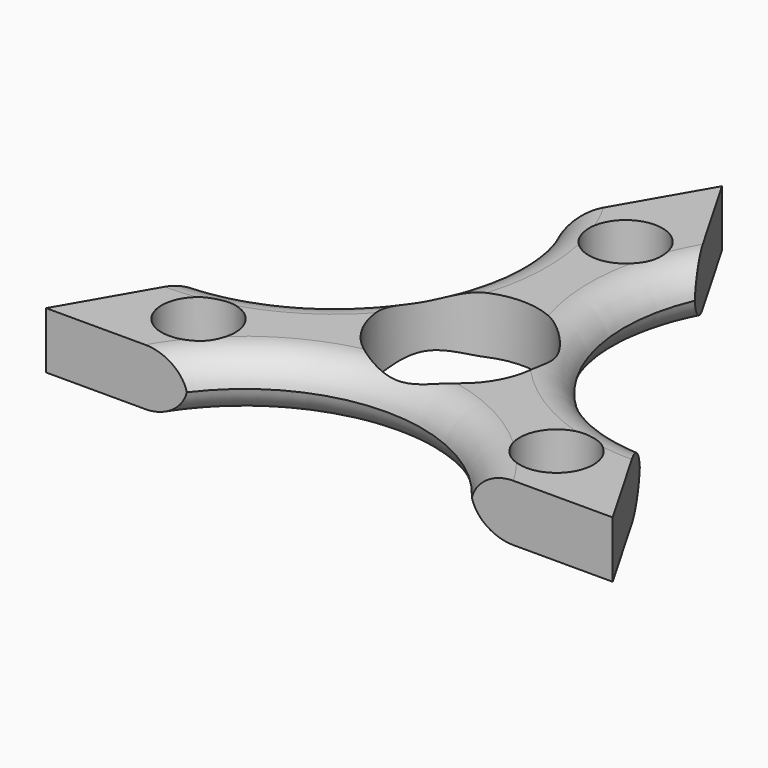
from build123d import *

# Parameters (mm, degrees)
F0_R         = 5.2
F0_R_2       = 11
F1_DEPTH     = 8
F2_T2_ANGLE  = 163.5880718536
F2_T4_ANGLE  = 163.5880718536
F2_T6_ANGLE  = 163.5880718536
F2_T8_ANGLE  = 163.5880718536
F2_T10_ANGLE = 163.5880718536
F2_T12_ANGLE = 163.5880718536


# Not quite as in the source:
# - a fillet or chamfer that OpenCascade refuses, or shapes differently, is made with other operations: its cross-section is extruded or revolved along the edge and cut away or added


with BuildPart() as f1:
    # F0 (on Top) → F1 (new body)
    with BuildSketch(Plane.XY):
        with BuildLine():
            Line((10, 28.4363744997), (0, 45.7568825754))
            Line((0, 45.7568825754), (-10, 28.4363744997))
            ThreePointArc((-10, 28.4363744997), (-11.3397459622, 6.115866424), (-30, -6.2046416517))
            Line((-30, -6.2046416517), (-40, -23.5251497274))
            Line((-40, -23.5251497274), (-20, -23.5251497274))
            ThreePointArc((-20, -23.5251497274), (0, -13.5251497274), (20, -23.5251497274))
            Line((20, -23.5251497274), (40, -23.5251497274))
            Line((40, -23.5251497274), (30, -6.2046416517))
            ThreePointArc((30, -6.2046416517), (11.3397459622, 6.115866424), (10, 28.4363744997))
        make_face()
        with Locations((-25.2775681357, -15.0251497274)):
            Circle(F0_R, mode=Mode.SUBTRACT)
        with Locations((25.2775681357, -15.0251497274)):
            Circle(F0_R, mode=Mode.SUBTRACT)
        with Locations((0, -0.4311389598)):
            Circle(F0_R_2, mode=Mode.SUBTRACT)
        with Locations((0, 28.7568825754)):
            Circle(F0_R, mode=Mode.SUBTRACT)
    extrude(amount=F1_DEPTH)

    # F2: fillet of radius 5 on 6 edges, made by hand

    # F2_s1 → F2_t2 (revolve, cut)
    with BuildSketch(Plane(origin=(-29.4179701652, 23.1546186531, 0), x_dir=(0, 0, 1), z_dir=(-0.7857925171, 0.618490194, 0))):
        with BuildLine():
            ThreePointArc((3, 19.2239813561), (6.5355339059, 20.6884474501), (8, 24.2239813561))
            Line((8, 24.2239813561), (8, 19.2239813561))
            Line((8, 19.2239813561), (3, 19.2239813561))
        make_face()
    revolve(axis=Axis((-32.9903810568, 18.615866424, 8), (0, 0, -1)), revolution_arc=F2_T2_ANGLE, mode=Mode.SUBTRACT)

    # F2_s3 → F2_t4 (revolve, cut)
    with BuildSketch(Plane(origin=(34.8604405257, 13.9389723807, 0), x_dir=(0, 0, 1), z_dir=(0.9285244785, 0.3712711849, 0))):
        with BuildLine():
            ThreePointArc((3, 19.9630902024), (6.5355339059, 21.4275562964), (8, 24.9630902024))
            Line((8, 24.9630902024), (8, 19.9630902024))
            Line((8, 19.9630902024), (3, 19.9630902024))
        make_face()
    revolve(axis=Axis((32.9903810568, 18.615866424, 8), (0, 0, -1)), revolution_arc=F2_T4_ANGLE, mode=Mode.SUBTRACT)

    # F2_s5 → F2_t6 (revolve, cut)
    with BuildSketch(Plane(origin=(-5.4424703605, -37.7402994735, 0), x_dir=(0, 0, 1), z_dir=(-0.1427319614, -0.9897613789, 0))):
        with BuildLine():
            ThreePointArc((3, 19.5012298151), (6.5355339059, 20.9656959092), (8, 24.5012298151))
            Line((8, 24.5012298151), (8, 19.5012298151))
            Line((8, 19.5012298151), (3, 19.5012298151))
        make_face()
    revolve(axis=Axis((0, -38.5251497274, 8), (0, 0, -1)), revolution_arc=F2_T6_ANGLE, mode=Mode.SUBTRACT)

    # F2_s7 → F2_t8 (revolve, cut)
    with BuildSketch(Plane(origin=(-29.4179701652, 23.1546186531, 0), x_dir=(0, 0, 1), z_dir=(-0.7857925171, 0.618490194, 0))):
        with BuildLine():
            ThreePointArc((5, 19.2239813561), (1.4644660941, 20.6884474501), (0, 24.2239813561))
            Line((0, 24.2239813561), (0, 19.2239813561))
            Line((0, 19.2239813561), (5, 19.2239813561))
        make_face()
    revolve(axis=Axis((-32.9903810568, 18.615866424, 0), (0, 0, -1)), revolution_arc=F2_T8_ANGLE, mode=Mode.SUBTRACT)

    # F2_s9 → F2_t10 (revolve, cut)
    with BuildSketch(Plane(origin=(34.8604405257, 13.9389723807, 0), x_dir=(0, 0, 1), z_dir=(0.9285244785, 0.3712711849, 0))):
        with BuildLine():
            ThreePointArc((5, 19.9630902024), (1.4644660941, 21.4275562964), (0, 24.9630902024))
            Line((0, 24.9630902024), (0, 19.9630902024))
            Line((0, 19.9630902024), (5, 19.9630902024))
        make_face()
    revolve(axis=Axis((32.9903810568, 18.615866424, 0), (0, 0, -1)), revolution_arc=F2_T10_ANGLE, mode=Mode.SUBTRACT)

    # F2_s11 → F2_t12 (revolve, cut)
    with BuildSketch(Plane(origin=(-5.4424703605, -37.7402994735, 0), x_dir=(0, 0, 1), z_dir=(-0.1427319614, -0.9897613789, 0))):
        with BuildLine():
            ThreePointArc((5, 19.5012298151), (1.4644660941, 20.9656959092), (0, 24.5012298151))
            Line((0, 24.5012298151), (0, 19.5012298151))
            Line((0, 19.5012298151), (5, 19.5012298151))
        make_face()
    revolve(axis=Axis((0, -38.5251497274, 0), (0, 0, -1)), revolution_arc=F2_T12_ANGLE, mode=Mode.SUBTRACT)


solid = f1.part
